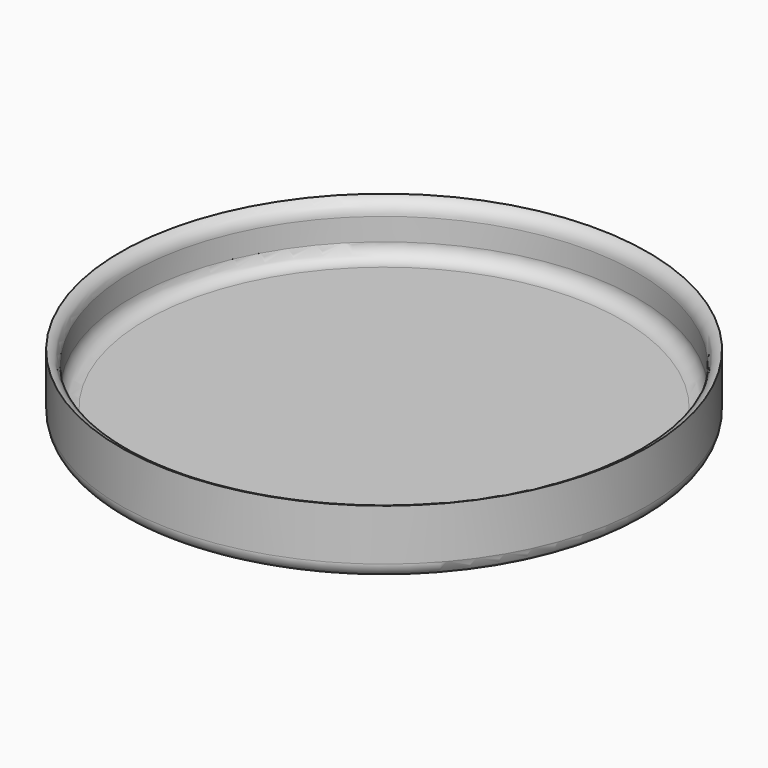
from build123d import *

# Parameters (mm, degrees)
F0_R     = 34.5
F1_DEPTH = 2
F0_R_2   = 36
F2_DEPTH = 9
F4_R     = 2


# Not quite as in the source:
# - a fillet or chamfer that OpenCascade refuses, or shapes differently, is made with other operations: its cross-section is extruded or revolved along the edge and cut away or added


with BuildPart() as f1:
    # F0 (on Top) → F1 (new body)
    with BuildSketch(Plane.XY):
        Circle(F0_R)
    extrude(amount=F1_DEPTH)

    # F0 (on Top) → F2 (join)
    with BuildSketch(Plane.XY):
        Circle(F0_R_2)
        Circle(F0_R, mode=Mode.SUBTRACT)
    extrude(amount=F2_DEPTH)

    # F3: fillet of radius 2 on 2 edges, made by hand

    # F3_s1 → F3_t2 (revolve)
    with BuildSketch(Plane.XZ):
        with BuildLine():
            ThreePointArc((34.5, 4), (33.9142135624, 2.5857864376), (32.5, 2))
            Line((32.5, 2), (34.5, 2))
            Line((34.5, 2), (34.5, 4))
        make_face()
    revolve(axis=Axis((0, 0, 2), (0, 0, 1)))

    # F3_s3 → F3_t4 (revolve, cut)
    with BuildSketch(Plane.XZ):
        with BuildLine():
            ThreePointArc((36, 9), (34.9188611699, 8.2882531983), (34.5, 7.0635083269))
            Line((34.5, 7.0635083269), (34.5, 9))
            Line((34.5, 9), (36, 9))
        make_face()
    revolve(axis=Axis((0, 0, 9), (0, 0, 1)), mode=Mode.SUBTRACT)

    # F4
    f4_edges = [f1.edges().sort_by_distance(p)[0] for p in [
        (-36, 0, 0),
    ]]
    fillet(f4_edges, radius=F4_R)


solid = f1.part
